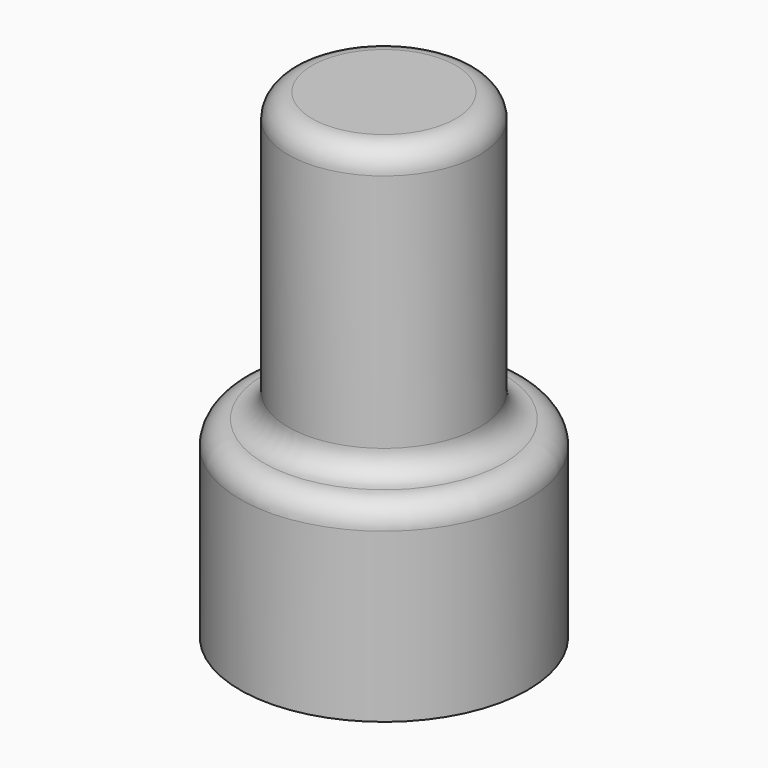
from build123d import *

# Parameters (mm, degrees)
F0_R     = 20
F1_DEPTH = 60
F0_R_2   = 30
F2_DEPTH = 40
F3_R     = 5
F4_R     = 5
F5_R     = 4.99999


# Not quite as in the source:
# - a fillet or chamfer is up to 0.001 mm smaller than in the source, because OpenCascade refuses the exact size


with BuildPart() as f1:
    # F0 (on Top) → F1 (new body)
    with BuildSketch(Plane.XY):
        Circle(F0_R)
    extrude(amount=F1_DEPTH)

    # F0 (on Top) → F2 (join)
    with BuildSketch(Plane.XY):
        Circle(F0_R_2)
        Circle(F0_R, mode=Mode.SUBTRACT)
        Circle(F0_R)
    extrude(amount=-F2_DEPTH)

    # F3
    f3_edges = [f1.edges().sort_by_distance(p)[0] for p in [
        (-20, 0, 60),
    ]]
    fillet(f3_edges, radius=F3_R)

    # F4
    f4_edges = [f1.edges().sort_by_distance(p)[0] for p in [
        (-30, 0, 0),
    ]]
    fillet(f4_edges, radius=F4_R)

    # F5 (radius 5 in the source; OpenCascade refuses exactly that, so slightly less here)
    f5_edges = [f1.edges().sort_by_distance(p)[0] for p in [
        (-20, 0, 0),
    ]]
    fillet(f5_edges, radius=F5_R)


solid = f1.part
